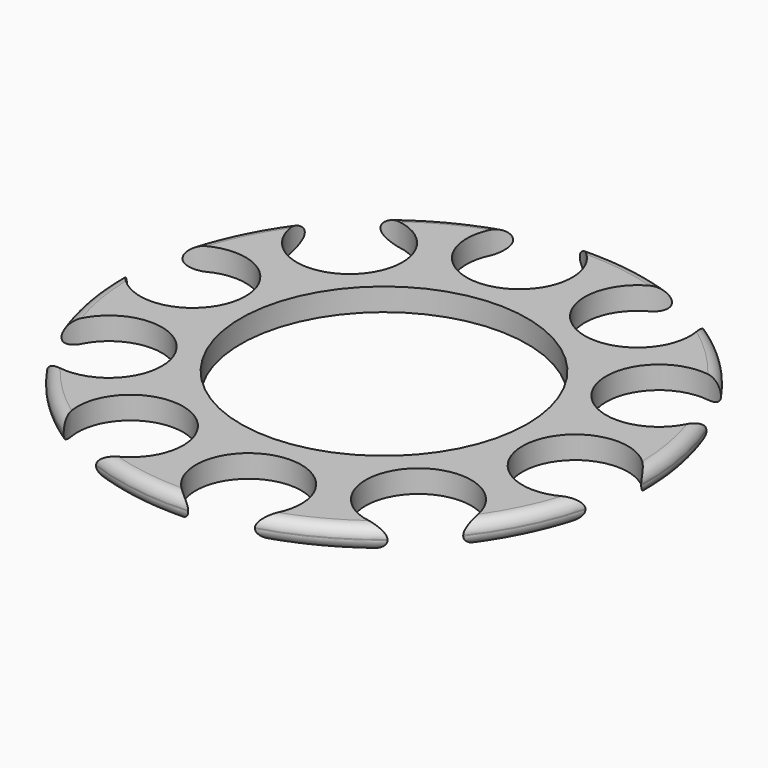
from build123d import *

# Parameters (mm, degrees)
F0_R     = 17.5
F0_R_2   = 9.5
F1_DEPTH = 1.5
F2_R     = 3.5
F3_DEPTH = 25
F4_R     = 0.7242640687


with BuildPart() as f1:
    # F0 (on Top) → F1 (new body)
    with BuildSketch(Plane.XY):
        Circle(F0_R)
        Circle(F0_R_2, mode=Mode.SUBTRACT)
    extrude(amount=F1_DEPTH)

    # F2 (on face) → F3 (cut)
    with BuildSketch(Plane.XY.offset(1.5)):
        with Locations((-10.3832991676, 10.1211214001)):
            Circle(F2_R)
        with Locations((-14.3493113799, 2.085009094)):
            Circle(F2_R)
        with Locations((-12.8343743603, -6.7475058192)):
            Circle(F2_R)
        with Locations((-6.4171425593, -13.0027028488)):
            Circle(F2_R)
        with Locations((2.4512195886, -14.2913093357)):
            Circle(F2_R)
        with Locations((10.3832991676, -10.1211214001)):
            Circle(F2_R)
        with Locations((14.3493113799, -2.085009094)):
            Circle(F2_R)
        with Locations((12.8343743603, 6.7475058192)):
            Circle(F2_R)
        with Locations((6.4171425593, 13.0027028488)):
            Circle(F2_R)
        with Locations((-2.4512195886, 14.2913093357)):
            Circle(F2_R)
    extrude(amount=-F3_DEPTH, mode=Mode.SUBTRACT)

    # F4
    f4_edges = [f1.edges().sort_by_distance(p)[0] for p in [
        (-17.248132, -2.958368, 1.5),
        (-17.248132, -2.958368, 0),
        (17.248132, 2.958368, 0),
        (17.248132, 2.958368, 1.5),
        (12.215147, 12.531568, 0),
        (12.215147, 12.531568, 1.5),
        (2.51639, 17.318134, 0),
        (2.51639, 17.318134, 1.5),
        (-8.143542, 15.489762, 0),
        (-8.143542, 15.489762, 1.5),
        (-15.692917, 7.744827, 0),
        (-15.692917, 7.744827, 1.5),
        (-12.215147, -12.531568, 1.5),
        (-12.215147, -12.531568, 0),
        (-2.51639, -17.318134, 1.5),
        (-2.51639, -17.318134, 0),
        (8.143542, -15.489762, 1.5),
        (8.143542, -15.489762, 0),
        (15.692917, -7.744827, 1.5),
        (15.692917, -7.744827, 0),
    ]]
    fillet(f4_edges, radius=F4_R)


solid = f1.part
